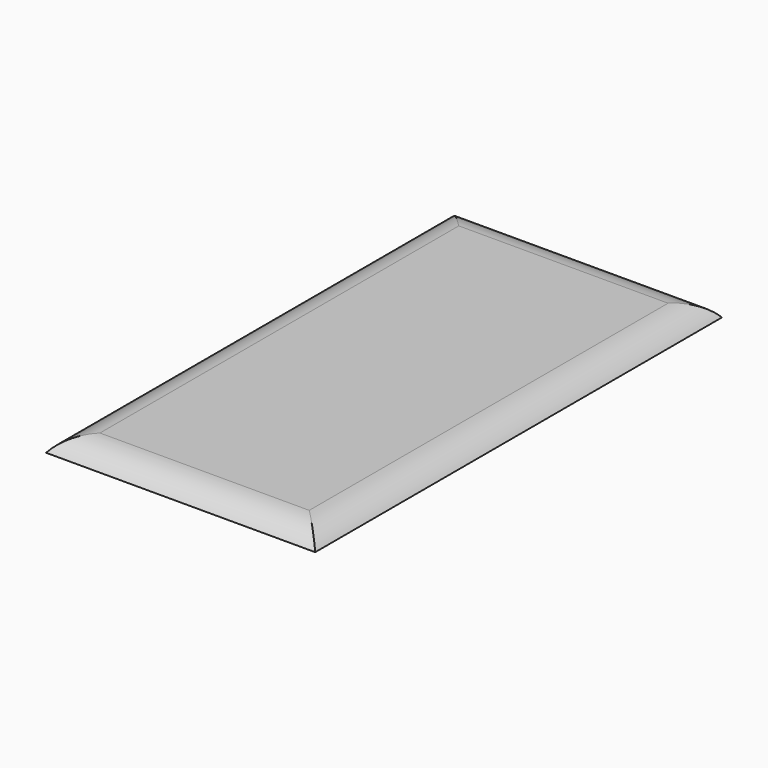
from build123d import *

# Parameters (mm, degrees)
F0_W        = 36
F0_H        = 68
F1_DEPTH    = 2
F2_T1_DEPTH = 88
F2_T3_DEPTH = 56


# Not quite as in the source:
# - a fillet or chamfer that OpenCascade refuses, or shapes differently, is made with other operations: its cross-section is extruded or revolved along the edge and cut away or added


with BuildPart() as f1:
    # F0 (on Top) → F1 (new body)
    with BuildSketch(Plane.XY):
        with Locations((18, 34)):
            Rectangle(F0_W, F0_H)
    extrude(amount=F1_DEPTH)

    # F2: fillet of radius 5 on 4 edges, made by hand

    # F2_s2 → F2_t1 (cut)
    with BuildSketch(Plane.XZ.offset(-78)):
        with BuildLine():
            ThreePointArc((36, 0), (34.2360679775, 1.472135955), (32, 2))
            Line((32, 2), (36, 2))
            Line((36, 2), (36, 0))
        make_face()
        with BuildLine():
            ThreePointArc((0, 0), (1.7639320225, 1.472135955), (4, 2))
            Line((4, 2), (0, 2))
            Line((0, 2), (0, 0))
        make_face()
    extrude(amount=F2_T1_DEPTH, mode=Mode.SUBTRACT)

    # F2_s4 → F2_t3 (cut)
    with BuildSketch(Plane.YZ.offset(-10)):
        with BuildLine():
            ThreePointArc((0, 0), (1.7639320225, 1.472135955), (4, 2))
            Line((4, 2), (0, 2))
            Line((0, 2), (0, 0))
        make_face()
        with BuildLine():
            ThreePointArc((68, 0), (66.2360679775, 1.472135955), (64, 2))
            Line((64, 2), (68, 2))
            Line((68, 2), (68, 0))
        make_face()
    extrude(amount=F2_T3_DEPTH, mode=Mode.SUBTRACT)


solid = f1.part
